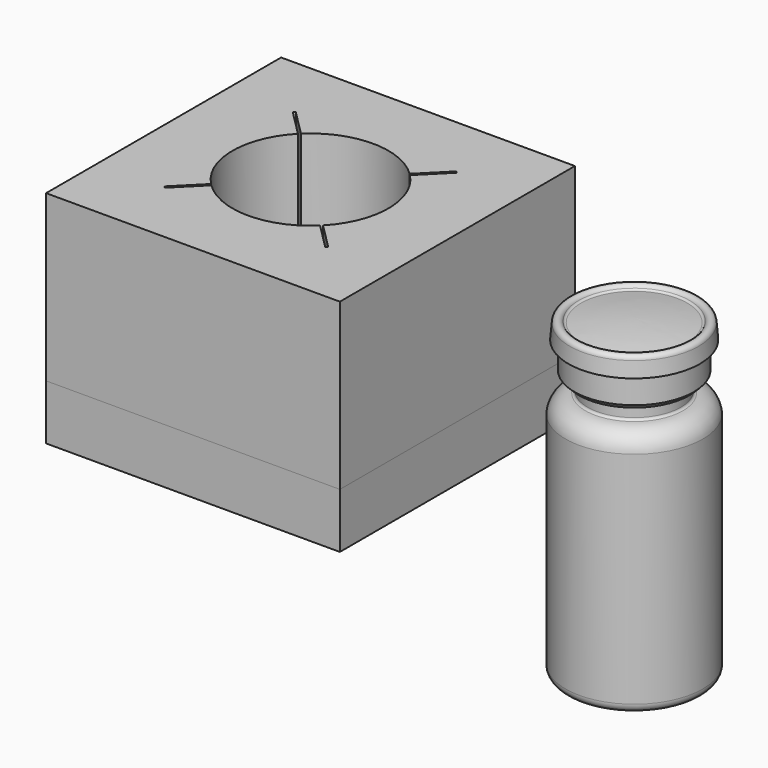
from build123d import *

# Parameters (mm, degrees)
F0_W     = 50.8
F0_H     = 50.8
F1_DEPTH = 28.575
F2_W     = 50.8
F2_H     = 50.8
F3_DEPTH = 9.525


# Not quite as in the source:
# - ends of sketch curves that miss each other by under 0.0002 mm in the source are joined


with BuildPart() as f1:
    # F0 (on Top) → F1 (new body)
    with BuildSketch(Plane.XY):
        with Locations((-21.9615258, 1.8580354)):
            Rectangle(F0_W, F0_H)
        with BuildLine():
            ThreePointArc((-31.3582782013, 11.5421633096), (-21.9615258, 15.3517854), (-12.5647733987, 11.5421633096))
            Line((-12.5647733987, 11.5421633096), (-8.074279, 16.0326324))
            ThreePointArc((-8.074279, 16.0326324), (-7.9298691961, 15.8896791745), (-7.7869234772, 15.7452620149))
            Line((-7.7869234772, 15.7452620149), (-12.2773948, 11.2547908))
            ThreePointArc((-12.2773948, 11.2547908), (-8.4677758, 1.8580354), (-12.2773978904, -7.5387170013))
            Line((-12.2773978904, -7.5387170013), (-7.7869288, -12.0292114))
            ThreePointArc((-7.7869288, -12.0292114), (-7.9298756108, -12.1736147892), (-8.074286225, -12.3165542255))
            Line((-8.074286225, -12.3165542255), (-12.5647704, -7.8260956))
            ThreePointArc((-12.5647704, -7.8260956), (-21.9615258, -11.6357146), (-31.3582782013, -7.8260925096))
            Line((-31.3582782013, -7.8260925096), (-35.8487472, -12.3165616))
            ThreePointArc((-35.8487472, -12.3165616), (-35.9931695745, -12.1736212039), (-36.1361154255, -12.029204175))
            Line((-36.1361154255, -12.029204175), (-31.6456314, -7.53872))
            ThreePointArc((-31.6456314, -7.53872), (-35.4552758, 1.8580354), (-31.6456413921, 11.2548004956))
            Line((-31.6456413921, 11.2548004956), (-36.1361228, 15.7452568))
            ThreePointArc((-36.1361228, 15.7452568), (-35.9931759892, 15.8896855892), (-35.8487524149, 16.0326377228))
            Line((-35.8487524149, 16.0326377228), (-31.3582782013, 11.5421633096))
        make_face(mode=Mode.SUBTRACT)
    extrude(amount=F1_DEPTH)


with BuildPart() as f3:
    # F2 (on face) → F3 (new body)
    with BuildSketch(Plane(origin=(0, 0, 0), x_dir=(1, 0, 0), z_dir=(0, 0, -1))):
        with Locations((-21.9615258, -1.8580354)):
            Rectangle(F2_W, F2_H)
    extrude(amount=F3_DEPTH)


with BuildPart() as f5:
    # F4 (on Front) → F5 (revolve)
    with BuildSketch(Plane.XZ):
        with BuildLine():
            Line((35.4933504, 26.97099), (35.4933504, -27.25801))
            Line((35.4933504, -27.25801), (45.7740004, -27.25801))
            ThreePointArc((45.7740004, -27.25801), (46.8965324151, -26.7930420151), (47.3615004, -25.67051))
            Line((47.3615004, -25.67051), (47.3615004, 12.37869))
            ThreePointArc((47.3615004, 12.37869), (46.2571032279, 14.627915971), (43.9342782618, 15.5677037122))
            ThreePointArc((43.9342782618, 15.5677037122), (43.6586666515, 15.6866290767), (43.5451504, 15.9645096))
            Line((43.5451504, 15.9645096), (43.5451504, 18.23974))
            Line((43.5451504, 18.23974), (45.0120004, 18.23974))
            Line((45.0120004, 18.23974), (45.8057504, 19.03349))
            Line((45.8057504, 19.03349), (45.8057504, 23.64359))
            Line((45.8057504, 23.64359), (46.8535004, 23.64359))
            Line((46.8535004, 23.64359), (46.6257894, 26.2464296))
            ThreePointArc((46.6257894, 26.2464296), (45.954733078, 26.9619169371), (45.1009053301, 26.4789899736))
            ThreePointArc((45.1009053301, 26.4789899736), (44.9278136613, 26.2836367625), (44.6708278714, 26.2380238884))
            ThreePointArc((44.6708278714, 26.2380238884), (40.096198354, 26.781168636), (35.4933504, 26.97099))
        make_face()
    revolve(axis=Axis((35.4933504, 0, -0.14351), (0, 0, -1)))


solid = Compound([f1.part, f3.part, f5.part])
